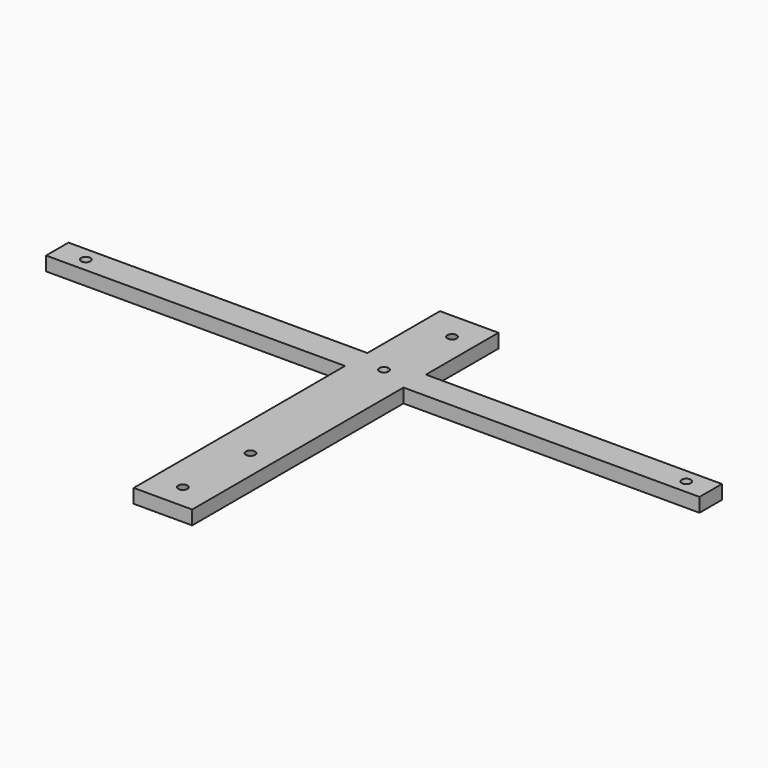
from build123d import *

# Parameters (mm, degrees)
F0_W     = 64.0446986989
F0_H     = 6
F0_R     = 1
F0_W_2   = 63.4251574627
F1_DEPTH = 3


# Not quite as in the source:
# - a feature names something its author has since deleted; it is built from what else it names


with BuildPart() as f1:
    # F0 (on Top) → F1 (new body)
    with BuildSketch(Plane.XY):
        Polygon((-7.5510093011, -42.2321148217), (-1.289947, -42.2321148217), (4.9791345373, -42.2321148217), (4.9791345373, 14.358856), (-1.595708, 14.358856), (-7.5510093011, 14.358856), align=None)
        Polygon((-0.297832, -36.78021), (-0.289947, -36.905543), (-0.297832, -37.030876), (-0.321364, -37.154233), (-0.360171, -37.273667), (-0.41364, -37.387296), (-0.48093, -37.493328), (-0.560978, -37.59009), (-0.652523, -37.676056), (-0.75412, -37.749871), (-0.864168, -37.81037), (-0.98093, -37.856599), (-1.102566, -37.88783), (-1.227157, -37.90357), (-1.352738, -37.90357), (-1.477328, -37.88783), (-1.598964, -37.856599), (-1.715726, -37.81037), (-1.825774, -37.749871), (-1.927371, -37.676056), (-2.018916, -37.59009), (-2.098964, -37.493328), (-2.166254, -37.387296), (-2.219724, -37.273667), (-2.25853, -37.154233), (-2.282062, -37.030876), (-2.289947, -36.905543), (-2.282062, -36.78021), (-2.25853, -36.656853), (-2.219724, -36.537418), (-2.166254, -36.423789), (-2.098964, -36.317758), (-2.018916, -36.220996), (-1.927371, -36.13503), (-1.825774, -36.061215), (-1.715726, -36.000716), (-1.598964, -35.954486), (-1.477328, -35.923256), (-1.352738, -35.907516), (-1.227157, -35.907516), (-1.102566, -35.923256), (-0.98093, -35.954486), (-0.864168, -36.000716), (-0.75412, -36.061215), (-0.652523, -36.13503), (-0.560978, -36.220996), (-0.48093, -36.317758), (-0.41364, -36.423789), (-0.360171, -36.537418), (-0.321364, -36.656853), align=None, mode=Mode.SUBTRACT)
        Polygon((0.834477, -20.078598), (0.842362, -20.203931), (0.834477, -20.329264), (0.810945, -20.452621), (0.772138, -20.572056), (0.718669, -20.685685), (0.651379, -20.791716), (0.571331, -20.888478), (0.479786, -20.974444), (0.378189, -21.048259), (0.268141, -21.108758), (0.151379, -21.154988), (0.029743, -21.186218), (-0.094848, -21.201958), (-0.220429, -21.201958), (-0.345019, -21.186218), (-0.466655, -21.154988), (-0.583417, -21.108758), (-0.693465, -21.048259), (-0.795062, -20.974444), (-0.886607, -20.888478), (-0.966655, -20.791716), (-1.033945, -20.685685), (-1.087415, -20.572056), (-1.126221, -20.452621), (-1.149753, -20.329264), (-1.157638, -20.203931), (-1.149753, -20.078598), (-1.126221, -19.955241), (-1.087415, -19.835807), (-1.033945, -19.722178), (-0.966655, -19.616146), (-0.886607, -19.519384), (-0.795062, -19.433418), (-0.693465, -19.359603), (-0.583417, -19.299104), (-0.466655, -19.252875), (-0.345019, -19.221644), (-0.220429, -19.205904), (-0.094848, -19.205904), (0.029743, -19.221644), (0.151379, -19.252875), (0.268141, -19.299104), (0.378189, -19.359603), (0.479786, -19.433418), (0.571331, -19.519384), (0.651379, -19.616146), (0.718669, -19.722178), (0.772138, -19.835807), (0.810945, -19.955241), align=None, mode=Mode.SUBTRACT)
        Polygon((-7.5510093011, 39.788339287), (-7.5510093011, 20.358856), (-1.595708, 20.358856), (4.9791345373, 20.358856), (4.9791345373, 28.8824737072), (4.9791345373, 39.788339287), (-1.289947, 39.788339287), align=None)
        Polygon((0.834477, 33.921402), (0.842362, 33.796069), (0.834477, 33.670736), (0.810945, 33.547379), (0.772138, 33.427944), (0.718669, 33.314315), (0.651379, 33.208284), (0.571331, 33.111522), (0.479786, 33.025556), (0.378189, 32.951741), (0.268141, 32.891242), (0.151379, 32.845012), (0.029743, 32.813782), (-0.094848, 32.798042), (-0.220429, 32.798042), (-0.345019, 32.813782), (-0.466655, 32.845012), (-0.583417, 32.891242), (-0.693465, 32.951741), (-0.795062, 33.025556), (-0.886607, 33.111522), (-0.966655, 33.208284), (-1.033945, 33.314315), (-1.087415, 33.427944), (-1.126221, 33.547379), (-1.149753, 33.670736), (-1.157638, 33.796069), (-1.149753, 33.921402), (-1.126221, 34.044759), (-1.087415, 34.164193), (-1.033945, 34.277822), (-0.966655, 34.383854), (-0.886607, 34.480616), (-0.795062, 34.566582), (-0.693465, 34.640397), (-0.583417, 34.700896), (-0.466655, 34.747125), (-0.345019, 34.778356), (-0.220429, 34.794096), (-0.094848, 34.794096), (0.029743, 34.778356), (0.151379, 34.747125), (0.268141, 34.700896), (0.378189, 34.640397), (0.479786, 34.566582), (0.571331, 34.480616), (0.651379, 34.383854), (0.718669, 34.277822), (0.772138, 34.164193), (0.810945, 34.044759), align=None, mode=Mode.SUBTRACT)
        with Locations((-39.5733586505, 17.358856)):
            Rectangle(F0_W, F0_H)
        with Locations((-65.4838681221, 17.358856)):
            Circle(F0_R, mode=Mode.SUBTRACT)
        with Locations((36.6917132686, 17.358856)):
            Rectangle(F0_W_2, F0_H)
        with Locations((63.1569251418, 17.358856)):
            Circle(F0_R, mode=Mode.SUBTRACT)
        with BuildLine():
            Line((-7.5510093011, 20.358856), (-7.5510093011, 14.358856))
            Line((-7.5510093011, 14.358856), (-1.595708, 14.358856))
            Line((-1.595708, 14.358856), (-1.595708, 16.358856))
            ThreePointArc((-1.595708, 16.358856), (-2.595708, 17.358856), (-1.595708, 18.358856))
            Line((-1.595708, 18.358856), (-1.595708, 20.358856))
            Line((-1.595708, 20.358856), (-7.5510093011, 20.358856))
        make_face()
        with BuildLine():
            Line((-1.595708, 14.358856), (4.9791345373, 14.358856))
            Line((4.9791345373, 14.358856), (4.9791345373, 20.358856))
            Line((4.9791345373, 20.358856), (-1.595708, 20.358856))
            Line((-1.595708, 20.358856), (-1.595708, 18.358856))
            ThreePointArc((-1.595708, 18.358856), (-0.8886012188, 18.0659627812), (-0.595708, 17.358856))
            ThreePointArc((-0.595708, 17.358856), (-0.8886012188, 16.6517492188), (-1.595708, 16.358856))
            Line((-1.595708, 16.358856), (-1.595708, 14.358856))
        make_face()
    extrude(amount=F1_DEPTH)


solid = f1.part
